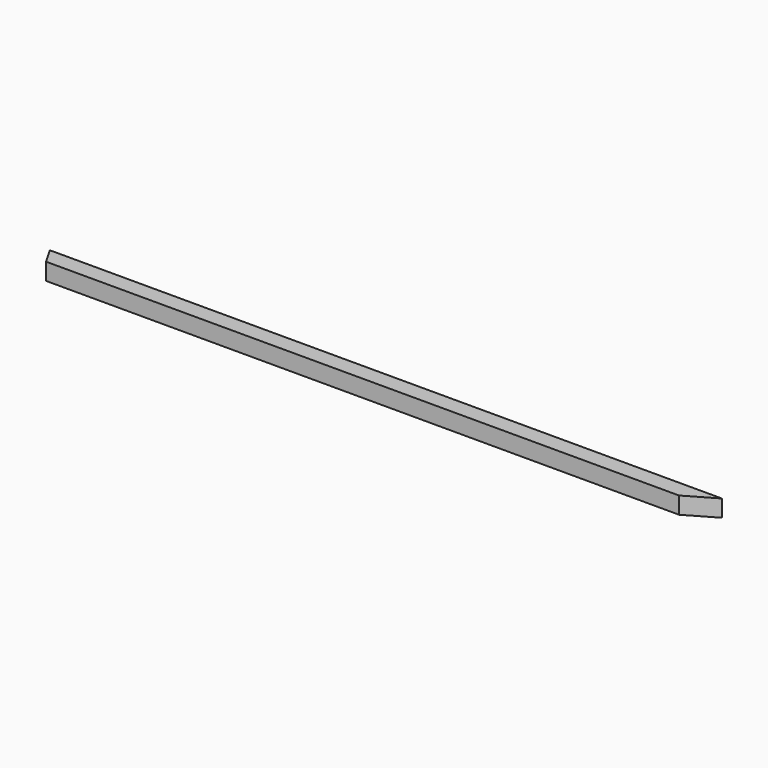
from build123d import *

# Parameters (mm, degrees)
F0_W        = 127
F0_H        = 3.175
F1_DEPTH    = 3.175
F2_T1_DEPTH = 23.6619672735
F3_T1_DEPTH = 35.0436157588


# Not quite as in the source:
# - a fillet or chamfer that OpenCascade refuses, or shapes differently, is made with other operations: its cross-section is extruded or revolved along the edge and cut away or added


with BuildPart() as f1:
    # F0 (on Front) → F1 (new body)
    with BuildSketch(Plane.XZ):
        with Locations((14.5824663341, 34.311569615)):
            Rectangle(F0_W, F0_H)
    extrude(amount=F1_DEPTH)

    # F2: chamfer of 2.286 x 3.9594681461 on 1 edges, made by hand

    # F2_s2 → F2_t1 (cut)
    with BuildSketch(Plane.XY.offset(22.4805859783)):
        Polygon((-48.9175336659, 0.7844681461), (-46.6315336659, -3.175), (-48.9175336659, -3.175), align=None)
    extrude(amount=F2_T1_DEPTH, mode=Mode.SUBTRACT)

    # F3: chamfer of 3.556 x 6.1591726717 on 1 edges, made by hand

    # F3_s2 → F3_t1 (cut)
    with BuildSketch(Plane.XY.offset(16.7897617356)):
        Polygon((78.0824663341, 0.381), (71.9232936624, -3.175), (78.0824663341, -3.175), align=None)
    extrude(amount=F3_T1_DEPTH, mode=Mode.SUBTRACT)


solid = f1.part
